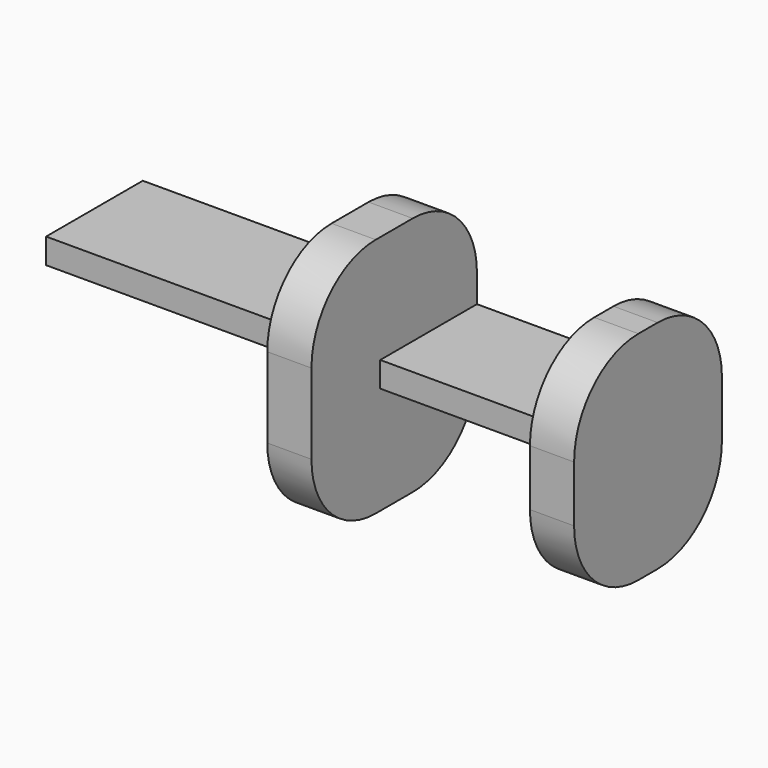
from build123d import *

# Parameters (mm, degrees)
F0_W     = 5.5
F0_H     = 27
F1_DEPTH = 23
F0_H_2   = 30
F2_DEPTH = 2.75
F3_R     = 10
F4_R     = 10
F5_W     = 15.0505993515
F5_H     = 3.1405385816
F6_DEPTH = 72.1


with BuildPart() as f1:
    # F0 (on Front) → F1 (new body)
    with BuildSketch(Plane.XZ):
        Rectangle(F0_W, F0_H)
    extrude(amount=F1_DEPTH)

    # F3
    f3_edges = [f1.edges().sort_by_distance(p)[0] for p in [
        (0, -23, -13.5),
        (0, -23, 13.5),
        (0, 0, -13.5),
        (0, 0, 13.5),
    ]]
    fillet(f3_edges, radius=F3_R)

    # F5 (on face) → F6 (join)
    with BuildSketch(Plane.YZ.offset(2.75)):
        with Locations((-7.5252996758, -0.032756303)):
            Rectangle(F5_W, F5_H)
    extrude(amount=-F6_DEPTH)


with BuildPart() as f1b:
    # F0 (on Front) → F1, piece 2 (new body)
    with BuildSketch(Plane.XZ):
        with Locations((-30.5, 0)):
            Rectangle(F0_W, F0_H_2)
    extrude(amount=F1_DEPTH)

    # F2 (add, symmetric): a face of the model
    f2_faces = [f1b.faces().sort_by_distance(p)[0] for p in [
        (-30.5, -23, 0),
    ]]
    extrude(f2_faces, amount=F2_DEPTH, both=True)

    # F4
    f4_edges = [f1b.edges().sort_by_distance(p)[0] for p in [
        (-30.5, 0, 15),
        (-30.5, 0, -15),
        (-30.5, -25.75, -15),
        (-30.5, -25.75, 15),
    ]]
    fillet(f4_edges, radius=F4_R)


solid = Compound([f1.part, f1b.part])
